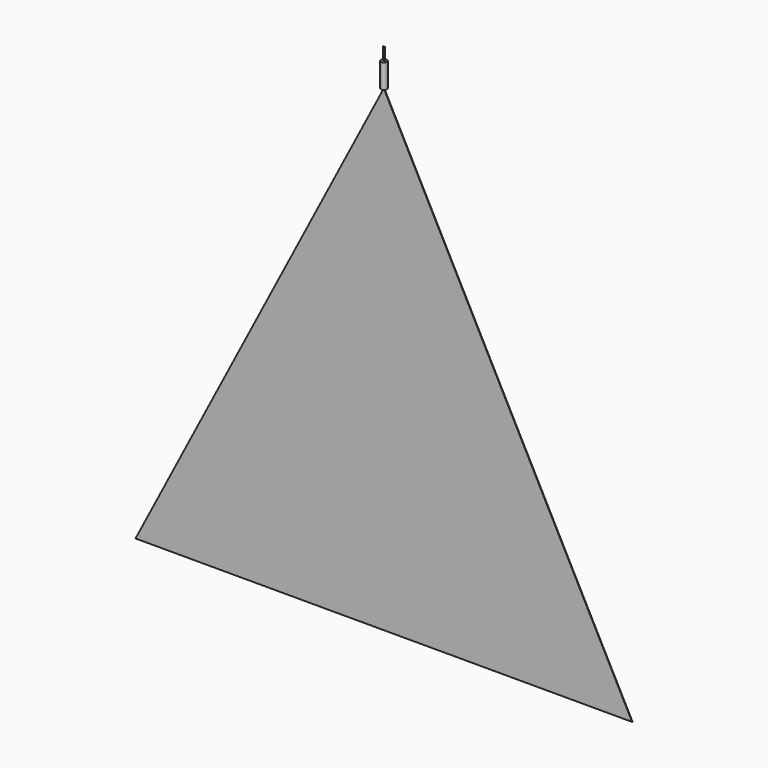
from build123d import *

# Parameters (mm, degrees)
F0_R     = 6
F1_DEPTH = 49.022
F2_R     = 0.508
F3_DEPTH = 25.4
F4_R     = 0.508
F5_DEPTH = 25.4
F7_DEPTH = 0.5
F9_DEPTH = 6.501


# Not quite as in the source:
# - a feature of the source that left no trace in its solid (it failed there, or was rolled back) is left out


with BuildPart() as f1:
    # F0 (on Top) → F1 (new body)
    with BuildSketch(Plane.XY):
        Circle(F0_R)
    extrude(amount=F1_DEPTH)

    # F8 (on face) → F9 (cut, through all)
    with BuildSketch(Plane.XZ.offset(0.5)):
        Polygon((108.475908637, 0), (38.0572463157, -73.1072899742), (366.4362130725, -703.9174159872), (858.39933024, -722.3438895265), align=None)
    extrude(amount=-F9_DEPTH, mode=Mode.SUBTRACT)


with BuildPart() as f3:
    # F2 (on face) → F3 (new body)
    with BuildSketch(Plane.XY.offset(49.022)):
        with Locations((-1.524, 0)):
            Circle(F2_R)
    extrude(amount=F3_DEPTH)


with BuildPart() as f5:
    # F4 (on face) → F5 (new body)
    with BuildSketch(Plane.XY.offset(49.022)):
        with Locations((1.524, 0)):
            Circle(F4_R)
    extrude(amount=F5_DEPTH)


with BuildPart() as f7:
    # F6 (on Front) → F7 (new body, symmetric)
    with BuildSketch(Plane.XZ):
        Polygon((502.4513171925, -965.2), (0, 0), (-502.4513171925, -965.2), align=None)
    extrude(amount=F7_DEPTH, both=True)


solid = Compound([f1.part, f3.part, f5.part, f7.part])
